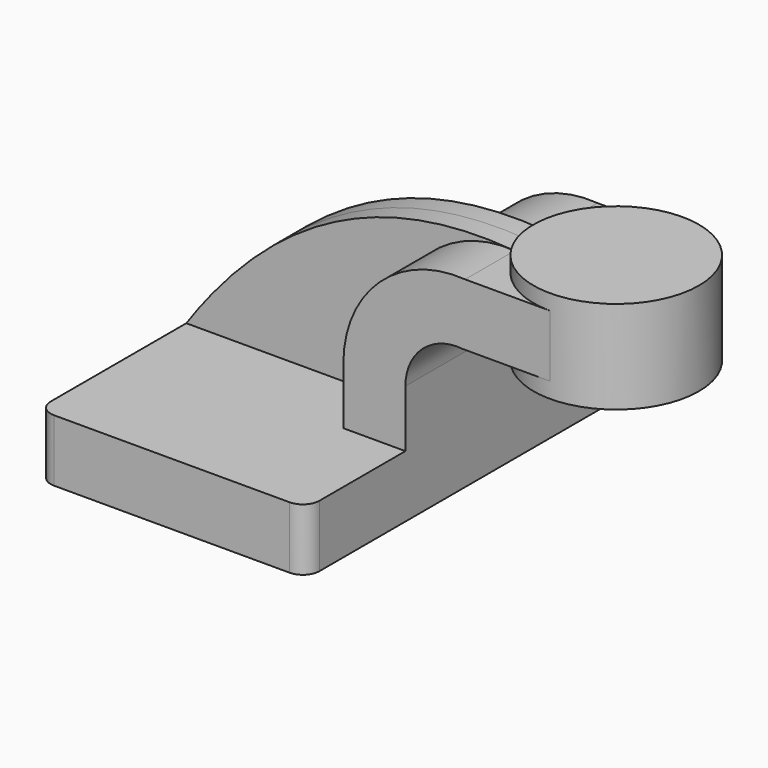
from build123d import *

# Parameters (mm, degrees)
F1_DEPTH = 63.5
F0_W     = 25.4
F0_H     = 19.05
F2_DEPTH = 25.4
F3_DEPTH = 6.35
F5_R     = 5.08


# Not quite as in the source:
# - a length typed as a fraction of an inch, garbled in the dataset ("3 / 203.2 mm" for 3/8 in), is restored


with BuildPart() as f1:
    # F0 (on Front) → F1 (new body, symmetric)
    with BuildSketch(Plane.XZ):
        Polygon((-41.275, -9.525), (41.275, -9.525), (41.275, 9.525), (22.225, 9.525), (-41.275, 9.525), align=None)
    extrude(amount=F1_DEPTH, both=True)

    # F0 (on Front) → F2 (join, symmetric)
    with BuildSketch(Plane.XZ):
        with BuildLine():
            Line((22.225, 9.525), (41.275, 9.525))
            Line((41.275, 9.525), (41.275, 27.1006073004))
            ThreePointArc((41.275, 27.1006073004), (46.5301853034, 38.9004022482), (58.8164375824, 42.8879))
            Line((58.8164375824, 42.8879), (60.325, 42.8879))
            Line((60.325, 42.8879), (60.325, 61.9379))
            Line((60.325, 61.9379), (59.6235930061, 61.9379))
            ThreePointArc((59.6235930061, 61.9379), (33.3449019193, 52.6558989318), (22.225, 27.1006073004))
            Line((22.225, 27.1006073004), (22.225, 9.525))
        make_face()
        with Locations((73.025, 52.4129)):
            Rectangle(F0_W, F0_H)
    extrude(amount=F2_DEPTH, both=True)

    # F0 (on Front) → F3 (join, symmetric)
    with BuildSketch(Plane.XZ):
        with BuildLine():
            add(Edge.make_bspline(
                [(59.6235930061, 61.9379), (21.0421923548, 65.1707053185), (-12.7928890288, 50.4826121032), (-41.275, 9.525)],
                knots=[0, 0, 0, 0, 113.6997720183, 113.6997720183, 113.6997720183, 113.6997720183], degree=3))
            Line((-41.275, 9.525), (22.225, 9.525))
            Line((22.225, 9.525), (22.225, 27.1006073004))
            ThreePointArc((22.225, 27.1006073004), (33.3449019193, 52.6558989318), (59.6235930061, 61.9379))
        make_face()
    extrude(amount=F3_DEPTH, both=True)

    # F0 (on Front) → F4 (revolve)
    with BuildSketch(Plane.XZ):
        Polygon((85.725, 66.675), (85.725, 61.9379), (85.725, 42.8879), (85.725, 38.1), (111.125, 38.1), (111.125, 66.675), align=None)
    revolve(axis=Axis((85.725, 0, 52.3875), (0, 0, -1)))

    # F5
    f5_edges = [f1.edges().sort_by_distance(p)[0] for p in [
        (41.275, -63.5, 0),
        (-41.275, -63.5, 0),
        (41.275, 63.5, 0),
        (-41.275, 63.5, 0),
    ]]
    fillet(f5_edges, radius=F5_R)


solid = f1.part
